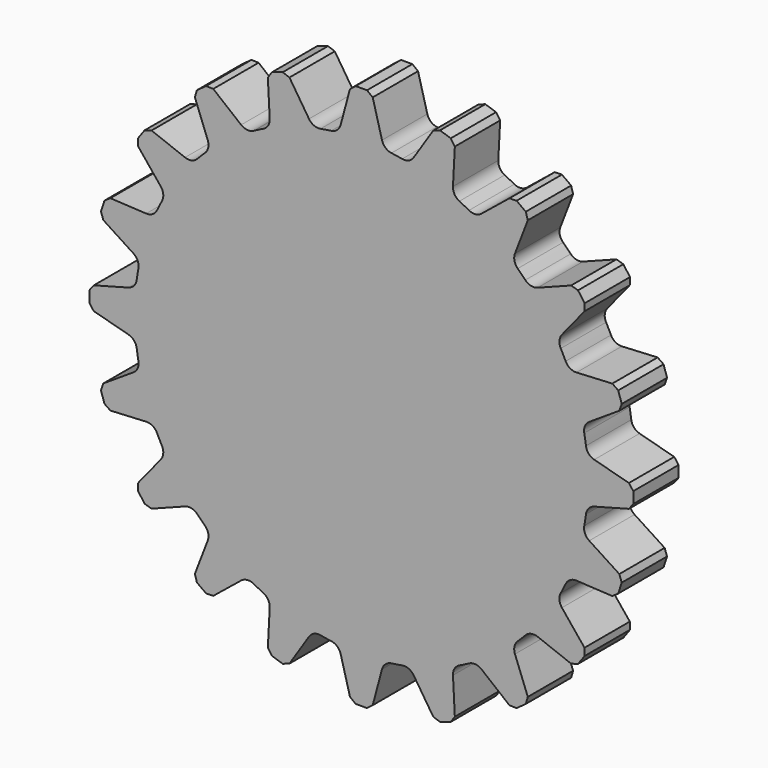
from build123d import *

# Parameters (mm, degrees)
F0_R            = 100
F1_DEPTH        = 25
F3_DEPTH        = 25
F3_COPIES_COUNT = 20
F4_SIZE         = 2
F5_R            = 5
F6_R            = 90
F7_DEPTH        = 10


# Not quite as in the source:
# - a pattern or mirror of a feature is missing from the dataset's text; its kind, count and spacing are read off the source's solid


with BuildPart() as f1:
    # F0 (on Front) → F1 (new body)
    with BuildSketch(Plane.XZ):
        Circle(F0_R)
    extrude(amount=F1_DEPTH)

    # F2 (on Front) → F3 (join)
    with BuildSketch(Plane.XZ):
        Polygon((-4.5, 120), (-9.9931095726, 99.4994359837), (9.9931095726, 99.4994359837), (4.5, 120), align=None)
    f3 = extrude(amount=F3_DEPTH)

    # F3_copies: F3 ×20 about axis
    f3_copies_axis = Axis((0, 0, 0), (0, 1, 0))
    for i in range(1, F3_COPIES_COUNT):
        add(f3.rotate(f3_copies_axis, i * 360 / F3_COPIES_COUNT))

    # F4
    f4_edges = [f1.edges().sort_by_distance(p)[0] for p in [
        (-4.5, -12.5, 120),
        (4.5, -12.5, 120),
        (-32.802285, -12.5, 115.517358),
        (115.517358, -12.5, 32.802285),
        (120, -12.5, 4.5),
        (120, -12.5, -4.5),
        (115.517358, -12.5, -32.802285),
        (112.736205, -12.5, -41.361794),
        (99.727073, -12.5, -66.893654),
        (94.437006, -12.5, -74.174807),
        (74.174807, -12.5, -94.437006),
        (66.893654, -12.5, -99.727073),
        (41.361794, -12.5, -112.736205),
        (32.802285, -12.5, -115.517358),
        (4.5, -12.5, -120),
        (-4.5, -12.5, -120),
        (-32.802285, -12.5, -115.517358),
        (-41.361794, -12.5, -112.736205),
        (-66.893654, -12.5, -99.727073),
        (-74.174807, -12.5, -94.437006),
        (-94.437006, -12.5, -74.174807),
        (-99.727073, -12.5, -66.893654),
        (-112.736205, -12.5, -41.361794),
        (-115.517358, -12.5, -32.802285),
        (-120, -12.5, -4.5),
        (-120, -12.5, 4.5),
        (-115.517358, -12.5, 32.802285),
        (-112.736205, -12.5, 41.361794),
        (-99.727073, -12.5, 66.893654),
        (-94.437006, -12.5, 74.174807),
        (-74.174807, -12.5, 94.437006),
        (-66.893654, -12.5, 99.727073),
        (32.802285, -12.5, 115.517358),
        (41.361794, -12.5, 112.736205),
        (66.893654, -12.5, 99.727073),
        (74.174807, -12.5, 94.437006),
        (94.437006, -12.5, 74.174807),
        (99.727073, -12.5, 66.893654),
        (112.736205, -12.5, 41.361794),
        (-41.361794, -12.5, 112.736205),
    ]]
    chamfer(f4_edges, length=F4_SIZE)

    # F5
    f5_edges = [f1.edges().sort_by_distance(p)[0] for p in [
        (-9.99311, -12.5, 99.499436),
        (9.99311, -12.5, 99.499436),
        (97.717628, -12.5, 21.243005),
        (99.499436, -12.5, 9.99311),
        (91.541546, -12.5, 40.251029),
        (86.370537, -12.5, 50.399706),
        (99.499436, -12.5, -9.99311),
        (97.717628, -12.5, -21.243005),
        (74.622932, -12.5, 66.568897),
        (66.568897, -12.5, 74.622932),
        (91.541546, -12.5, -40.251029),
        (86.370537, -12.5, -50.399706),
        (50.399706, -12.5, 86.370537),
        (40.251029, -12.5, 91.541546),
        (74.622932, -12.5, -66.568897),
        (66.568897, -12.5, -74.622932),
        (21.243005, -12.5, 97.717628),
        (50.399706, -12.5, -86.370537),
        (40.251029, -12.5, -91.541546),
        (-21.243005, -12.5, 97.717628),
        (21.243005, -12.5, -97.717628),
        (9.99311, -12.5, -99.499436),
        (-40.251029, -12.5, 91.541546),
        (-50.399706, -12.5, 86.370537),
        (-9.99311, -12.5, -99.499436),
        (-21.243005, -12.5, -97.717628),
        (-66.568897, -12.5, 74.622932),
        (-74.622932, -12.5, 66.568897),
        (-40.251029, -12.5, -91.541546),
        (-50.399706, -12.5, -86.370537),
        (-86.370537, -12.5, 50.399706),
        (-91.541546, -12.5, 40.251029),
        (-66.568897, -12.5, -74.622932),
        (-74.622932, -12.5, -66.568897),
        (-97.717628, -12.5, 21.243005),
        (-99.499436, -12.5, 9.99311),
        (-86.370537, -12.5, -50.399706),
        (-91.541546, -12.5, -40.251029),
        (-99.499436, -12.5, -9.99311),
        (-97.717628, -12.5, -21.243005),
    ]]
    fillet(f5_edges, radius=F5_R)

    # F6 (on face) → F7 (cut)
    with BuildSketch(Plane(origin=(0, 0, 0), x_dir=(-1, 0, 0), z_dir=(0, 1, 0))):
        Circle(F6_R)
    extrude(amount=-F7_DEPTH, mode=Mode.SUBTRACT)


solid = f1.part
